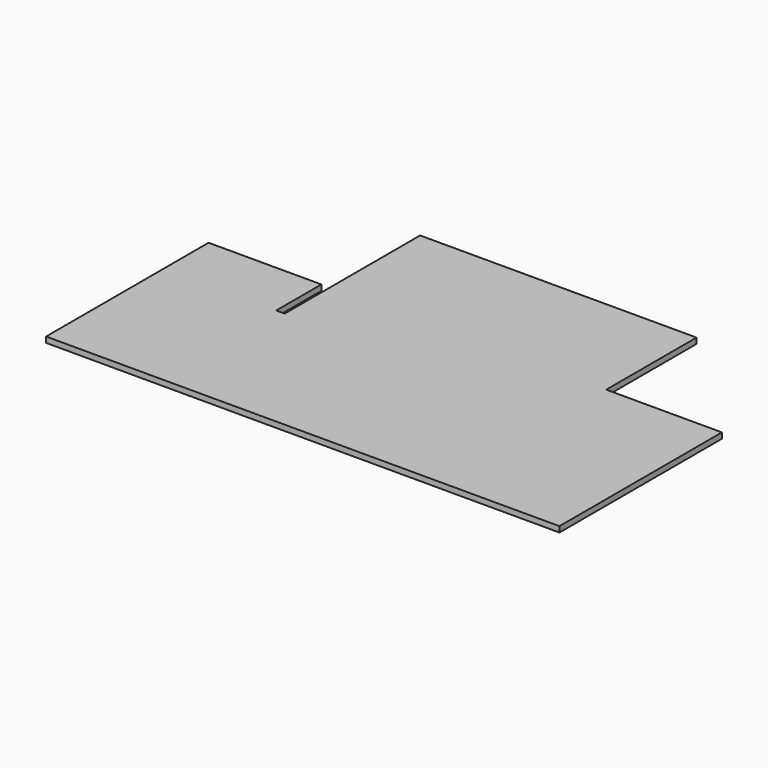
from build123d import *

# Parameters (mm, degrees)
F1_DEPTH = 1.5875


# Not quite as in the source:
# - a length typed as a fraction of an inch, garbled in the dataset ("3 / 203.2 mm" for 3/8 in), is restored


with BuildPart() as f1:
    # F0 (on Top) → F1 (new body, symmetric)
    with BuildSketch(Plane.XY):
        Polygon((-71.9991720523, 0), (-135.4991720523, 0), (-135.4991720523, -114.3), (153.4258279477, -114.3), (153.4258279477, 0), (88.3383279477, 0), (88.3383279477, 63.5), (-67.2366720523, 63.5), (-67.2366720523, -31.75), (-71.9991720523, -31.75), align=None)
    extrude(amount=F1_DEPTH, both=True)


solid = f1.part
